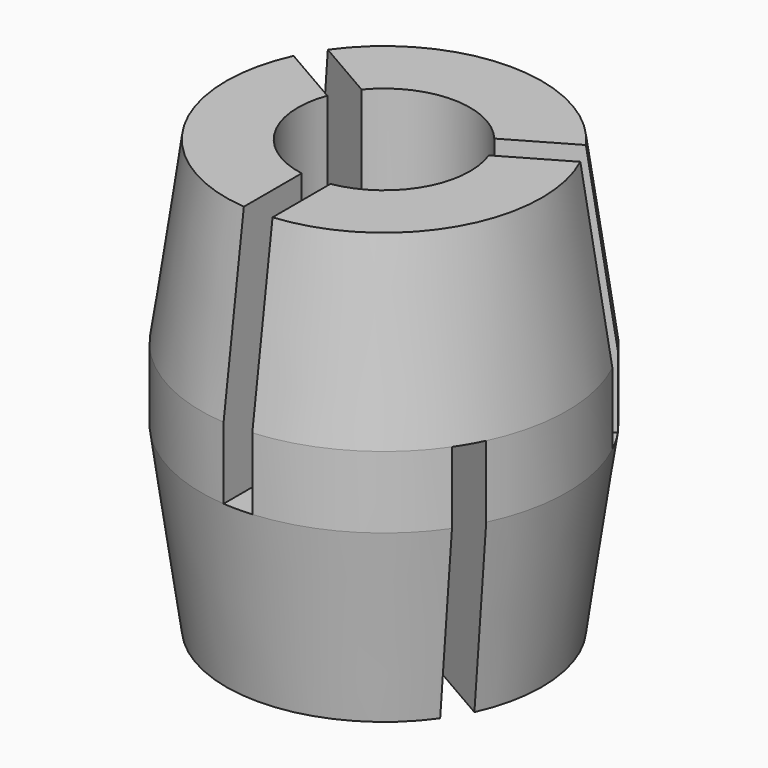
from build123d import *

# Parameters (mm, degrees)
F0_W     = 6.7567604338
F0_H     = 5
F3_DEPTH = 5
F6_DEPTH = 25
F7_DEPTH = 25


# Not quite as in the source:
# - a feature names something its author has since deleted; it is built from what else it names


with BuildPart() as f1:
    # F0 (on Front) → F1 (revolve)
    with BuildSketch(Plane.XZ):
        with Locations((9.3783802169, 15)):
            Rectangle(F0_W, F0_H)
    revolve(axis=Axis((0, 0, -3.2319817692), (0, 0, -1)))

    # F2 (on face) → F3 (cut, through all)
    with BuildSketch(Plane.XY.offset(17.5)):
        with BuildLine():
            ThreePointArc((1, 12.7175051313), (0, 12.7567604338), (-1, 12.7175051313))
            Line((-1, 12.7175051313), (-1, 5.9160797831))
            ThreePointArc((-1, 5.9160797831), (0, 6), (1, 5.9160797831))
            Line((1, 5.9160797831), (1, 12.7175051313))
        make_face()
        with BuildLine():
            Line((-4.623475383, 3.8240652953), (-10.5136825165, 7.2247779694))
            ThreePointArc((-10.5136825165, 7.2247779694), (-11.0476786056, 6.3783802169), (-11.5136825165, 5.4927271619))
            Line((-11.5136825165, 5.4927271619), (-5.623475383, 2.0920144878))
            ThreePointArc((-5.623475383, 2.0920144878), (-5.1961524227, 3), (-4.623475383, 3.8240652953))
        make_face()
        with BuildLine():
            Line((-5.623475383, -2.0920144878), (-11.5136825165, -5.4927271619))
            ThreePointArc((-11.5136825165, -5.4927271619), (-11.0476786056, -6.3783802169), (-10.5136825165, -7.2247779694))
            Line((-10.5136825165, -7.2247779694), (-4.623475383, -3.8240652953))
            ThreePointArc((-4.623475383, -3.8240652953), (-5.1961524227, -3), (-5.623475383, -2.0920144878))
        make_face()
        with BuildLine():
            Line((-1, -5.9160797831), (-1, -12.7175051313))
            ThreePointArc((-1, -12.7175051313), (0, -12.7567604338), (1, -12.7175051313))
            Line((1, -12.7175051313), (1, -5.9160797831))
            ThreePointArc((1, -5.9160797831), (0, -6), (-1, -5.9160797831))
        make_face()
        with BuildLine():
            ThreePointArc((10.5136825165, -7.2247779694), (11.0476786056, -6.3783802169), (11.5136825165, -5.4927271619))
            Line((11.5136825165, -5.4927271619), (5.623475383, -2.0920144878))
            ThreePointArc((5.623475383, -2.0920144878), (5.1961524227, -3), (4.623475383, -3.8240652953))
            Line((4.623475383, -3.8240652953), (10.5136825165, -7.2247779694))
        make_face()
        with BuildLine():
            ThreePointArc((11.5136825165, 5.4927271619), (11.0476786056, 6.3783802169), (10.5136825165, 7.2247779694))
            Line((10.5136825165, 7.2247779694), (4.623475383, 3.8240652953))
            ThreePointArc((4.623475383, 3.8240652953), (5.1961524227, 3), (5.623475383, 2.0920144878))
            Line((5.623475383, 2.0920144878), (11.5136825165, 5.4927271619))
        make_face()
    extrude(amount=-F3_DEPTH, mode=Mode.SUBTRACT)


with BuildPart() as f4:
    # F0 (on Front) → F4 (revolve)
    with BuildSketch(Plane.XZ):
        Polygon((6, 30), (6, 17.5), (12.7567604338, 17.5), (11, 30), align=None)
    revolve(axis=Axis((0, 0, -3.2319817692), (0, 0, -1)))


with BuildPart() as f4b:
    # F0 (on Front) → F4, piece 2 (revolve)
    with BuildSketch(Plane.XZ):
        Polygon((6, 12.5), (6, 0), (11, 0), (12.7567604338, 12.5), align=None)
    revolve(axis=Axis((0, 0, -3.2319817692), (0, 0, -1)))


with BuildPart() as f1_1:
    add(f1.part)

    # F5: union F4b, F4
    add(f4b.part)
    add(f4.part)

    # F6 (cut): faces of the model
    f6_faces = [f1_1.faces().sort_by_distance(p)[0] for p in [
        (0, -9.3578583369, 17.5),
        (8.1041430447, 4.6789291684, 17.5),
        (-8.1041430447, 4.6789291684, 17.5),
    ]]
    extrude(f6_faces, amount=-F6_DEPTH, mode=Mode.SUBTRACT)

    # F7 (cut): faces of the model
    f7_faces = [f1_1.faces().sort_by_distance(p)[0] for p in [
        (8.1041430447, -4.6789291684, 12.5),
        (0, 9.3578583369, 12.5),
        (-8.1041430447, -4.6789291684, 12.5),
    ]]
    extrude(f7_faces, amount=-F7_DEPTH, mode=Mode.SUBTRACT)


solid = f1_1.part
